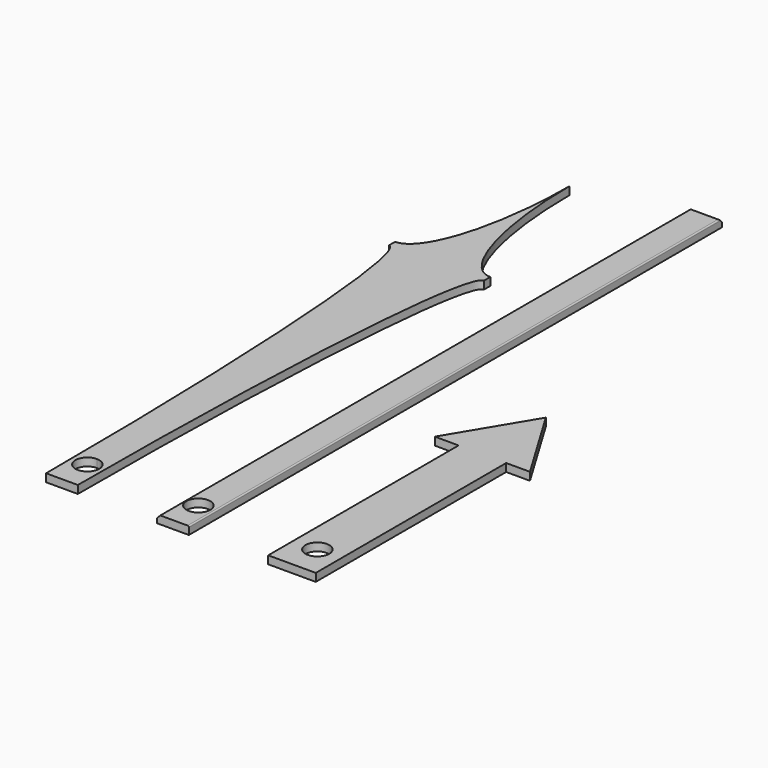
from build123d import *

# Parameters (mm, degrees)
F0_W        = 10
F0_H        = 2.5
F1_DEPTH    = 2.5
F2_W        = 10
F2_H        = 210
F2_R        = 3.75
F3_DEPTH    = 2.5
F4_R        = 3.75
F5_DEPTH    = 2.5
F6_SIZE     = 1
F7_T1_DEPTH = 211
F7_T3_DEPTH = 9.8284271247


# Not quite as in the source:
# - a fillet or chamfer that OpenCascade refuses, or shapes differently, is made with other operations: its cross-section is extruded or revolved along the edge and cut away or added


with BuildPart() as f1:
    # F0 (on Top) → F1 (new body)
    with BuildSketch(Plane.XY):
        with BuildLine():
            Line((0, 6.25), (0, 0))
            Line((0, 0), (5, 0))
            add(Edge.make_bspline(
                [(15, 147.5), (5, 147.5), (5, 0)],
                knots=[3.1415926536, 3.1415926536, 3.1415926536, 4.7123889804, 4.7123889804, 4.7123889804], degree=2, weights=[1, 0.7071067812, 1]))
            Line((15, 147.5), (5, 147.5))
            Line((5, 147.5), (5, 150))
            Line((5, 150), (0, 150))
            Line((0, 150), (0, 13.75))
            ThreePointArc((0, 13.75), (2.6516504294, 12.6516504294), (3.75, 10))
            ThreePointArc((3.75, 10), (2.6516504294, 7.3483495706), (0, 6.25))
        make_face()
        with Locations((10, 148.75)):
            Rectangle(F0_W, F0_H)
        with BuildLine():
            Line((0, 200), (0, 150))
            Line((0, 150), (5, 150))
            Line((5, 150), (15, 150))
            add(Edge.make_bspline(
                [(0, 200), (0, 150), (15, 150)],
                knots=[4.7123889804, 4.7123889804, 4.7123889804, 6.2831853072, 6.2831853072, 6.2831853072], degree=2, weights=[1, 0.7071067812, 1]))
        make_face()
        with BuildLine():
            Line((-5, 0), (0, 0))
            Line((0, 0), (0, 6.25))
            ThreePointArc((0, 6.25), (-3.75, 10), (0, 13.75))
            Line((0, 13.75), (0, 150))
            Line((0, 150), (0, 200))
            add(Edge.make_bspline(
                [(-15, 150), (0, 150), (0, 200)],
                knots=[3.1415926536, 3.1415926536, 3.1415926536, 4.7123889804, 4.7123889804, 4.7123889804], degree=2, weights=[1, 0.7071067812, 1]))
            Line((-15, 150), (-15, 147.5))
            add(Edge.make_bspline(
                [(-5, 0), (-5, 147.5), (-15, 147.5)],
                knots=[1.5707963268, 1.5707963268, 1.5707963268, 3.1415926536, 3.1415926536, 3.1415926536], degree=2, weights=[1, 0.7071067812, 1]))
        make_face()
    extrude(amount=F1_DEPTH)


with BuildPart() as f3:
    # F2 (on Top) → F3 (new body)
    with BuildSketch(Plane.XY):
        with Locations((35, 105)):
            Rectangle(F2_W, F2_H)
        with Locations((35, 10)):
            Circle(F2_R, mode=Mode.SUBTRACT)
    extrude(amount=F3_DEPTH)

    # F6
    f6_edges = [f3.edges().sort_by_distance(p)[0] for p in [
        (35, 210, 2.5),
        (30, 105, 2.5),
    ]]
    chamfer(f6_edges, length=F6_SIZE)

    # F7: fillet of radius 0.4 on 2 edges, made by hand

    # F7_s2 → F7_t1 (cut)
    with BuildSketch(Plane.XZ.offset(-210)):
        with BuildLine():
            add(Edge.make_bspline(
                [(40, 2.1), (40, 2.5), (39.6, 2.5)],
                knots=[0, 0, 0, 1, 1, 1], degree=2, weights=[1, 1, 1]))
            Line((39.6, 2.5), (40, 2.5))
            Line((40, 2.5), (40, 2.1))
        make_face()
    extrude(amount=F7_T1_DEPTH, mode=Mode.SUBTRACT)

    # F7_s4 → F7_t3 (cut)
    with BuildSketch(Plane.YZ.offset(30.5857864376)):
        with BuildLine():
            add(Edge.make_bspline(
                [(209.1171572875, 2.3828427125), (209, 2.5), (208.8343145751, 2.5)],
                knots=[0, 0, 0, 1, 1, 1], degree=2, weights=[1, 1, 1]))
            Line((208.8343145751, 2.5), (209, 2.5))
            Line((209, 2.5), (209.1171572875, 2.3828427125))
        make_face()
    extrude(amount=F7_T3_DEPTH, mode=Mode.SUBTRACT)


with BuildPart() as f5:
    # F4 (on Top) → F5 (new body)
    with BuildSketch(Plane.XY):
        Polygon((65, 75), (65, 0), (80, 0), (80, 75), (87.5, 75), (72.5, 100), (57.5, 75), align=None)
        with Locations((72.5, 10)):
            Circle(F4_R, mode=Mode.SUBTRACT)
    extrude(amount=F5_DEPTH)


solid = Compound([f1.part, f3.part, f5.part])
